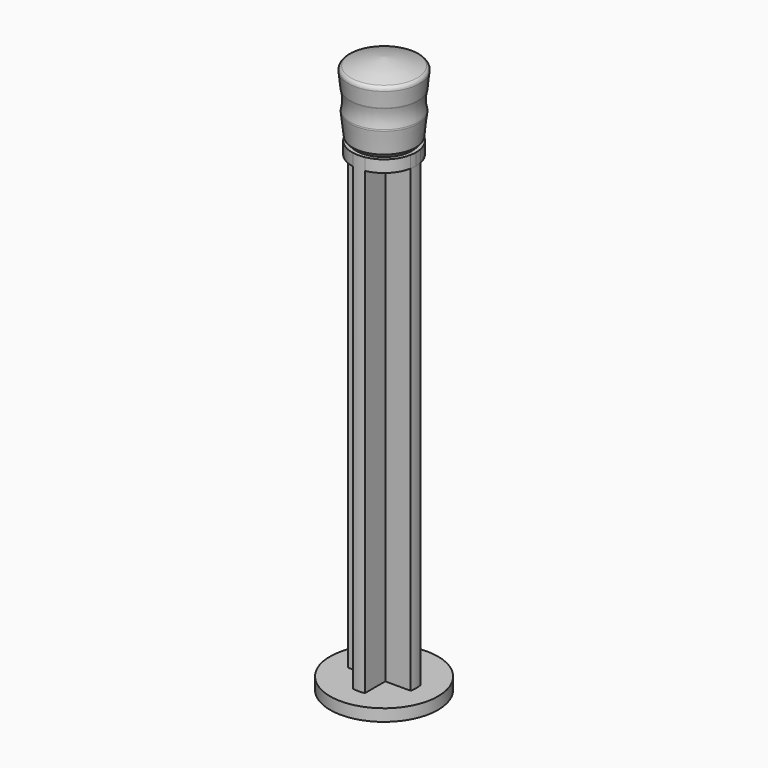
from build123d import *

# Parameters (mm, degrees)
F1_DEPTH = 59
F0_R     = 6.75
F2_DEPTH = 1.5
F4_DEPTH = 1.5
F7_R     = 0.5


with BuildPart() as f1:
    # F0 (on Top) → F1 (new body)
    with BuildSketch(Plane.XY):
        with BuildLine():
            Line((0.75, -0.75), (3.9290584114, -0.75))
            ThreePointArc((3.9290584114, -0.75), (4, 0), (3.9290584114, 0.75))
            Line((3.9290584114, 0.75), (0.75, 0.75))
            Line((0.75, 0.75), (0.75, 3.9290584114))
            ThreePointArc((0.75, 3.9290584114), (0, 4), (-0.75, 3.9290584114))
            Line((-0.75, 3.9290584114), (-0.75, 0.75))
            Line((-0.75, 0.75), (-3.9290584114, 0.75))
            ThreePointArc((-3.9290584114, 0.75), (-4, 0), (-3.9290584114, -0.75))
            Line((-3.9290584114, -0.75), (-0.75, -0.75))
            Line((-0.75, -0.75), (-0.75, -3.9290584114))
            ThreePointArc((-0.75, -3.9290584114), (0, -4), (0.75, -3.9290584114))
            Line((0.75, -3.9290584114), (0.75, -0.75))
        make_face()
    extrude(amount=F1_DEPTH)

    # F0 (on Top) → F2 (join)
    with BuildSketch(Plane.XY):
        Circle(F0_R)
        with BuildLine():
            ThreePointArc((3.9290584114, 0.75), (4, 0), (3.9290584114, -0.75))
            Line((3.9290584114, -0.75), (0.75, -0.75))
            Line((0.75, -0.75), (0.75, -3.9290584114))
            ThreePointArc((0.75, -3.9290584114), (0, -4), (-0.75, -3.9290584114))
            Line((-0.75, -3.9290584114), (-0.75, -0.75))
            Line((-0.75, -0.75), (-3.9290584114, -0.75))
            ThreePointArc((-3.9290584114, -0.75), (-4, 0), (-3.9290584114, 0.75))
            Line((-3.9290584114, 0.75), (-0.75, 0.75))
            Line((-0.75, 0.75), (-0.75, 3.9290584114))
            ThreePointArc((-0.75, 3.9290584114), (0, 4), (0.75, 3.9290584114))
            Line((0.75, 3.9290584114), (0.75, 0.75))
            Line((0.75, 0.75), (3.9290584114, 0.75))
        make_face(mode=Mode.SUBTRACT)
    extrude(amount=F2_DEPTH)

    # F3 (on face) → F4 (join)
    with BuildSketch(Plane.XY.offset(59)):
        with BuildLine():
            Line((0.75, 0.75), (3.9290584114, 0.75))
            ThreePointArc((3.9290584114, 0.75), (2.8284271247, 2.8284271247), (0.75, 3.9290584114))
            Line((0.75, 3.9290584114), (0.75, 0.75))
        make_face()
        with BuildLine():
            ThreePointArc((0.75, -3.9290584114), (2.8284271247, -2.8284271247), (3.9290584114, -0.75))
            Line((3.9290584114, -0.75), (0.75, -0.75))
            Line((0.75, -0.75), (0.75, -3.9290584114))
        make_face()
        with BuildLine():
            ThreePointArc((3.9290584114, -0.75), (3.9822251095, -0.376673834), (4, 0))
            ThreePointArc((4, 0), (3.9822251095, 0.376673834), (3.9290584114, 0.75))
            Line((3.9290584114, 0.75), (0.75, 0.75))
            Line((0.75, 0.75), (0.75, 3.9290584114))
            ThreePointArc((0.75, 3.9290584114), (0, 4), (-0.75, 3.9290584114))
            Line((-0.75, 3.9290584114), (-0.75, 0.75))
            Line((-0.75, 0.75), (-3.9290584114, 0.75))
            ThreePointArc((-3.9290584114, 0.75), (-4, 0), (-3.9290584114, -0.75))
            Line((-3.9290584114, -0.75), (-0.75, -0.75))
            Line((-0.75, -0.75), (-0.75, -3.9290584114))
            ThreePointArc((-0.75, -3.9290584114), (0, -4), (0.75, -3.9290584114))
            Line((0.75, -3.9290584114), (0.75, -0.75))
            Line((0.75, -0.75), (3.9290584114, -0.75))
        make_face()
        with BuildLine():
            Line((-0.75, 0.75), (-0.75, 3.9290584114))
            ThreePointArc((-0.75, 3.9290584114), (-2.8284271247, 2.8284271247), (-3.9290584114, 0.75))
            Line((-3.9290584114, 0.75), (-0.75, 0.75))
        make_face()
        with BuildLine():
            ThreePointArc((-3.9290584114, -0.75), (-2.8284271247, -2.8284271247), (-0.75, -3.9290584114))
            Line((-0.75, -3.9290584114), (-0.75, -0.75))
            Line((-0.75, -0.75), (-3.9290584114, -0.75))
        make_face()
    extrude(amount=F4_DEPTH)

    # F5 (on Front) → F6 (revolve)
    with BuildSketch(Plane.XZ):
        with BuildLine():
            Line((0, 69.7286576033), (0, 60.5))
            Line((0, 60.5), (3.5, 60.5))
            Line((3.5, 60.5), (3.9378246292, 61))
            Line((3.9378246292, 61), (4.25, 63.8117790222))
            ThreePointArc((4.25, 63.8117790222), (4.0865524412, 65.0321356952), (4.25, 66.2524923682))
            Line((4.25, 66.2524923682), (4.5, 68.5945898294))
            ThreePointArc((4.5, 68.5945898294), (2.2943533304, 69.3376184772), (0, 69.7286576033))
        make_face()
    revolve(axis=Axis((0, 0, 64.0703399479), (0, 0, 1)))

    # F7
    f7_edges = [f1.edges().sort_by_distance(p)[0] for p in [
        (-4.25, 0, 66.252492),
        (-4.25, 0, 63.811779),
        (-4.5, 0, 68.59459),
    ]]
    fillet(f7_edges, radius=F7_R)


solid = f1.part
